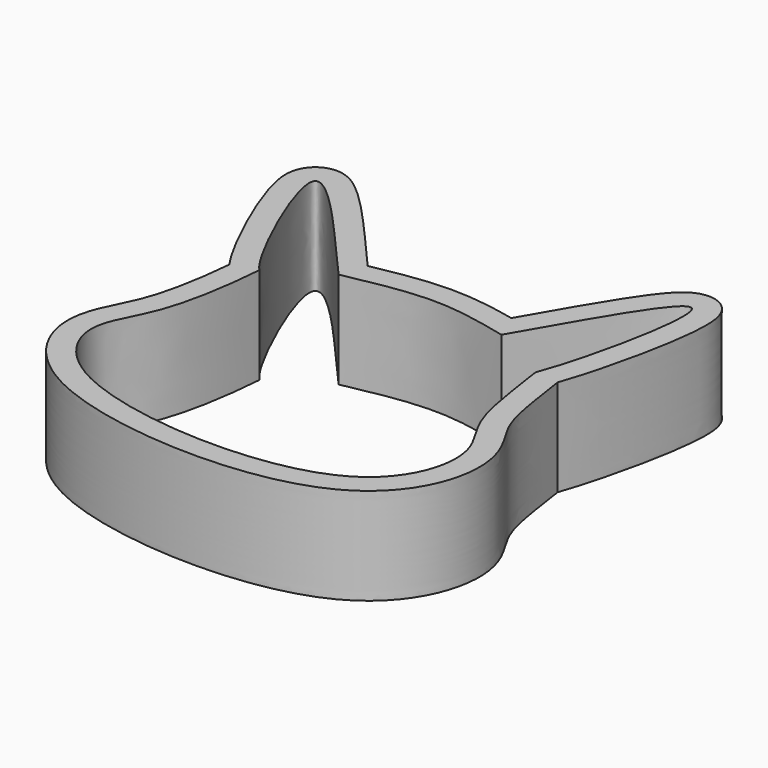
from build123d import *

# Parameters (mm, degrees)
F1_DEPTH = 26.162


# Not quite as in the source:
# - ends of sketch curves that miss each other by under 0.0002 mm in the source are joined
# - the dataset's text gives a spline's control points without its knots; the knots are read off the source's solid


with BuildPart() as f1:
    # F0 (on Top) → F1 (new body)
    with BuildSketch(Plane.XY):
        with BuildLine():
            add(Edge.make_bspline(
                [(-44.6860015518, 9.491417242), (-44.749575219, 9.5804256398), (-45.0524187399, 10.0093596103), (-45.8306026541, 11.1677582588), (-47.0458152965, 13.1497335365), (-48.5677804551, 15.852907993), (-50.1370771556, 18.8310918191), (-51.7267084692, 22.0215949113), (-53.3041855073, 25.3552671548), (-54.8349850059, 28.7607149006), (-56.2837104163, 32.166376281), (-57.6149274357, 35.5027429316), (-58.5972962812, 38.1712821381), (-59.2901935806, 40.2127667404), (-59.7593095455, 41.6929921589), (-60.1738199584, 43.1203276443), (-60.529489055, 44.4970475305), (-60.8213860842, 45.8324901102), (-61.0416924399, 47.1492620762), (-61.153403734, 48.2694208253), (-61.1772355316, 49.2288081315), (-61.1490556885, 50.0012448565), (-61.0522229548, 50.8539179365), (-60.8450298998, 51.8207778635), (-60.5183918295, 52.7493638887), (-60.1051195715, 53.5629095056), (-59.5665143071, 54.4094506867), (-58.6512150708, 55.4455312189), (-57.2098771495, 56.4383562858), (-55.6518810436, 57.0205934663), (-54.2099193721, 57.225112506), (-52.9819714323, 57.1815230494), (-51.9605562108, 57.001644524), (-51.1015447309, 56.7518761913), (-50.1132927783, 56.3694926186), (-49.0785310837, 55.8386584371), (-47.978488207, 55.1469281289), (-46.9359648501, 54.3951861603), (-45.9074869074, 53.5783581952), (-44.8710813836, 52.6934674951), (-43.4639636118, 51.4228837079), (-41.643723285, 49.6689620535), (-39.356642503, 47.331517145), (-36.9861221356, 44.8067557426), (-34.5602419367, 42.1460487186), (-32.1120020646, 39.4043717532), (-29.6770101711, 36.6388632662), (-26.4978736575, 32.9980915016), (-23.7392404848, 29.8252227516), (-21.9349590127, 27.7771817472), (-21.4940632775, 27.2793794942)],
                knots=[0.0427366583, 0.0427366583, 0.0427366583, 0.0427366583, 0.046875, 0.0625, 0.09375, 0.125, 0.15625, 0.1875, 0.21875, 0.25, 0.28125, 0.3125, 0.34375, 0.359375, 0.375, 0.390625, 0.40625, 0.421875, 0.4375, 0.453125, 0.4609375, 0.46875, 0.4765625, 0.484375, 0.4921875, 0.49609375, 0.5, 0.5078125, 0.515625, 0.5234375, 0.53125, 0.5390625, 0.546875, 0.5546875, 0.5625, 0.578125, 0.59375, 0.609375, 0.625, 0.640625, 0.65625, 0.6875, 0.71875, 0.75, 0.78125, 0.8125, 0.84375, 0.875, 0.9375, 0.9586784307, 0.9586784307, 0.9586784307, 0.9586784307], degree=3))
            add(Edge.make_bspline(
                [(-44.6860015518, 9.491417242), (-44.7714587328, 8.5588844477), (-45.054729235, 5.729834862), (-45.5688717525, 1.7173045707), (-46.2291374504, -2.281475048), (-46.8020728186, -5.2327262782), (-47.453573502, -8.0757528339), (-48.0604246314, -10.3023886994), (-48.5801769934, -11.9632050157), (-48.986068229, -13.1419654416), (-49.402352404, -14.2343377596), (-49.8507955536, -15.3054749749), (-50.3260446504, -16.3624900954), (-50.9906310093, -17.7662110369), (-51.8680929259, -19.5328935979), (-52.94926045, -21.7513120916), (-53.9881555406, -24.1578348121), (-54.7251799667, -26.397164995), (-55.1527930953, -28.3537523503), (-55.3678711892, -29.897506101), (-55.4537094577, -31.5156118644), (-55.3958177261, -33.1480658565), (-55.1979961143, -34.7830007969), (-54.7498118021, -36.9565262121), (-53.8499213198, -39.6422852284), (-52.2455192049, -42.7648791696), (-50.1339341643, -45.7462592521), (-47.5287652746, -48.552842567), (-44.4390179196, -51.156474213), (-41.4630772728, -53.1364465265), (-38.8417568776, -54.5952247955), (-36.0560661564, -55.9665546844), (-32.3339679057, -57.4928823796), (-27.5201746, -59.0627847159), (-20.7060946817, -60.8222250113), (-11.5786496644, -62.4087790119), (-0.1184123121, -63.305570292), (9.4460871539, -63.1579022595), (16.8667802613, -62.4529048796), (22.260244257, -61.6129031451), (27.4275208365, -60.4388172665), (31.5029178906, -59.1551847992), (34.5997414274, -57.9210687792), (36.4618895177, -57.056237693), (37.9028865359, -56.3039379862), (39.3128351743, -55.507622562), (40.99014051, -54.4407958458), (42.8561056483, -53.0618098635), (45.1502439825, -51.1033009579), (47.6516944087, -48.4587666757), (50.074726048, -45.0616359319), (51.9390606973, -41.5289861654), (53.2734892687, -37.9398978069), (54.1094350035, -34.3620188952), (54.4141860324, -31.4361788114), (54.4317392047, -29.1509678332), (54.3487462263, -27.7489942159), (54.2257046303, -26.6460712686), (54.0638172146, -25.5528148301), (53.6843622101, -23.7052640492), (52.9117679058, -21.2932329813), (51.7755103604, -18.7772744955), (50.5853352774, -16.6024551467), (49.6460734467, -15.0178052408), (48.9647570483, -13.8528552927), (48.4947905691, -13.0228326511), (48.070179522, -12.2285496877), (47.7562062634, -11.5902430885), (47.52857638, -11.0876969666), (47.3045466074, -10.5633910739), (47.0347062087, -9.8743282806), (46.7250831902, -8.9871528663), (46.3305441698, -7.7211416471), (45.869523594, -5.9770669701), (45.3590679025, -3.6166154191), (44.7177943587, -0.1077562981), (44.0130011423, 4.5352171987), (43.3992563303, 8.7560177557), (43.1003050473, 10.7371979302)],
                knots=[0.01507724, 0.01507724, 0.01507724, 0.01507724, 0.03125, 0.0625, 0.078125, 0.09375, 0.109375, 0.125, 0.1328125, 0.140625, 0.1484375, 0.15625, 0.1640625, 0.171875, 0.1875, 0.203125, 0.21875, 0.234375, 0.2421875, 0.25, 0.2578125, 0.265625, 0.2734375, 0.28125, 0.296875, 0.3125, 0.328125, 0.34375, 0.359375, 0.375, 0.3828125, 0.390625, 0.40625, 0.421875, 0.4375, 0.46875, 0.5, 0.53125, 0.546875, 0.5625, 0.578125, 0.59375, 0.6015625, 0.609375, 0.61328125, 0.6171875, 0.625, 0.6328125, 0.640625, 0.65625, 0.671875, 0.6875, 0.703125, 0.71875, 0.734375, 0.7421875, 0.75, 0.75390625, 0.7578125, 0.765625, 0.78125, 0.796875, 0.8125, 0.828125, 0.8359375, 0.84375, 0.8515625, 0.859375, 0.86328125, 0.8671875, 0.875, 0.8828125, 0.890625, 0.90625, 0.921875, 0.9375, 0.96875, 0.9934474336, 0.9934474336, 0.9934474336, 0.9934474336], degree=3))
            add(Edge.make_bspline(
                [(17.0948199289, 27.5811851309), (17.3516980768, 28.0266651427), (18.7023463682, 30.3734896214), (20.7120732251, 33.8862678296), (23.0972391532, 38.0115388324), (24.9028570602, 41.0948052745), (26.7060437795, 44.1154295497), (28.4890917464, 47.0233023559), (30.2365654481, 49.7709440487), (31.9375109277, 52.315448058), (33.3137972729, 54.2372186799), (34.3999821727, 55.6464206514), (35.2144233238, 56.6400085254), (36.0410166478, 57.5735502314), (36.9025212037, 58.4546162773), (37.8418556695, 59.2951713671), (38.7567737632, 59.9750271508), (39.6506442472, 60.5021083179), (40.4356444542, 60.8783579615), (41.3744275123, 61.2114817146), (42.5061208536, 61.4513206911), (43.8441619699, 61.5129549967), (45.0825356113, 61.3264916181), (46.0690251608, 61.0066909632), (46.7825494862, 60.6863472807), (47.4466554348, 60.2965778926), (48.2296671509, 59.7201990102), (49.0130721399, 58.9405135352), (49.679757904, 58.0232985478), (50.1485368788, 57.1687351534), (50.5914587849, 56.1198108796), (50.9196674499, 54.950882646), (51.1403965751, 53.662025441), (51.258360798, 52.4074548294), (51.3061935822, 51.1419586848), (51.2991483209, 49.8404083996), (51.22767631, 48.0398317463), (51.0350987094, 45.6504916269), (50.6637304879, 42.5597999245), (50.1690825093, 39.2756743956), (49.5664891354, 35.8402689292), (48.870520287, 32.3024029977), (48.0954838853, 28.7141326684), (47.2554637404, 25.1291573088), (46.0671841423, 20.4258407194), (44.6703933432, 15.475058208), (43.5631323168, 12.0636441862), (43.1003050473, 10.7371979302)],
                knots=[0.0475766477, 0.0475766477, 0.0475766477, 0.0475766477, 0.0625, 0.125, 0.15625, 0.1875, 0.21875, 0.25, 0.28125, 0.3125, 0.34375, 0.359375, 0.375, 0.390625, 0.40625, 0.421875, 0.4375, 0.4453125, 0.453125, 0.4609375, 0.46875, 0.4765625, 0.484375, 0.48828125, 0.4921875, 0.49609375, 0.5, 0.5078125, 0.515625, 0.5234375, 0.53125, 0.546875, 0.5625, 0.578125, 0.59375, 0.609375, 0.625, 0.65625, 0.6875, 0.71875, 0.75, 0.78125, 0.8125, 0.84375, 0.875, 0.9375, 0.9818713836, 0.9818713836, 0.9818713836, 0.9818713836], degree=3))
            add(Edge.make_bspline(
                [(-21.4940632775, 27.2793794942), (-20.7163737185, 27.4332736325), (-17.9555834619, 27.9720073206), (-14.1596782955, 28.6516539359), (-10.1127846436, 29.2312517097), (-7.0603132973, 29.5759414392), (-3.99171785, 29.8085015488), (-1.4253932183, 29.8896225368), (0.6374769345, 29.8735657304), (2.675150489, 29.8022045167), (5.1731380833, 29.618994097), (8.0939715985, 29.2738064077), (11.8900600139, 28.6801725216), (14.8625779305, 28.075046182), (16.8713108878, 27.6309890842), (17.0948199289, 27.5811851309)],
                knots=[0.0757097712, 0.0757097712, 0.0757097712, 0.0757097712, 0.125, 0.25, 0.3125, 0.375, 0.4375, 0.5, 0.53125, 0.5625, 0.625, 0.6875, 0.75, 0.875, 0.8906983632, 0.8906983632, 0.8906983632, 0.8906983632], degree=3))
        make_face()
        with BuildLine():
            add(Edge.make_bspline(
                [(-38.1433868105, 11.5267410591), (-38.7537596189, 3.4828245995), (-41.3314101179, -16.7321506872), (-52.7794328493, -31.1088972219), (-37.8568871951, -57.0520258832), (40.8327495966, -61.2528548762), (51.2528494053, -26.370766866), (39.7129697653, -13.9097592998), (38.3323957365, 0), (36.5802033998, 11.3720705691)],
                knots=[0, 0, 0, 0, 0.1448695769, 0.2554040342, 0.3865498412, 0.6166556254, 0.7571395179, 0.8606899879, 1, 1, 1, 1], degree=3))
            add(Edge.make_bspline(
                [(-38.1433868105, 11.5267410591), (-42.7219017239, 15.800023075), (-71.2300231225, 77.8812617351), (-32.9644157931, 30.3545909851), (-23.7969066948, 20.3403197229)],
                knots=[0, 0, 0, 0, 0.49764484, 1, 1, 1, 1], degree=3))
            add(Edge.make_bspline(
                [(-23.7969066948, 20.3403197229), (-15.7005150993, 21.9772991395), (-0.1268987897, 25.1260709152), (13.6253498783, 21.8927202212), (20.2280972153, 20.3403197229)],
                knots=[0, 0, 0, 0, 0.5198787125, 1, 1, 1, 1], degree=3))
            add(Edge.make_bspline(
                [(20.2280972153, 20.3403197229), (28.0048781521, 33.5324146157), (53.2474486516, 80.9588749476), (41.4250702875, 24.3926507924), (36.5802033998, 11.3720705691)],
                knots=[0, 0, 0, 0, 0.4934126044, 1, 1, 1, 1], degree=3))
        make_face(mode=Mode.SUBTRACT)
    extrude(amount=F1_DEPTH)


solid = f1.part
